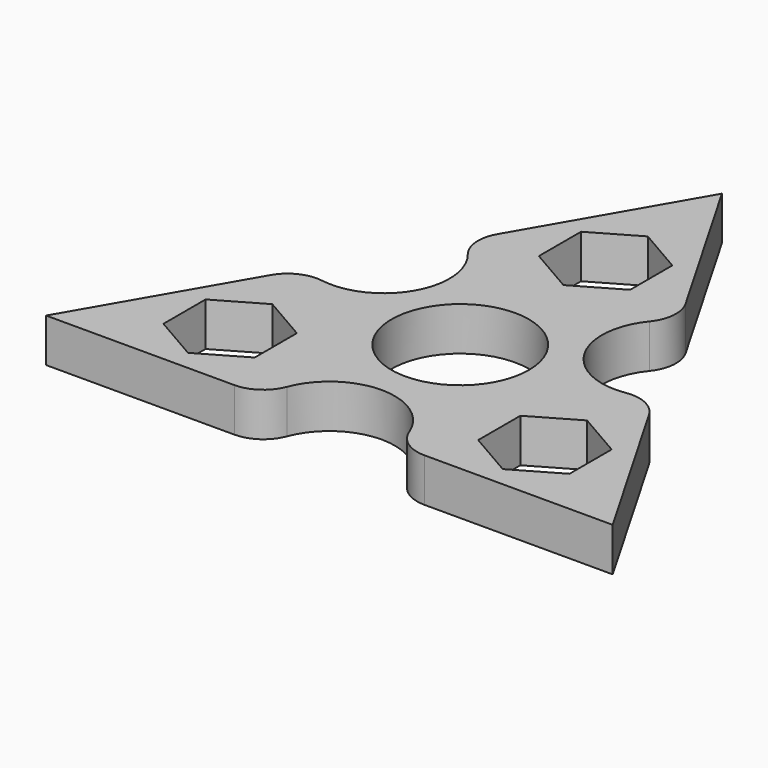
from build123d import *

# Parameters (mm, degrees)
F0_R     = 9.45
F1_DEPTH = 6
F2_R     = 5


with BuildPart() as f1:
    # F0 (on Top) → F1 (new body)
    with BuildSketch(Plane.XY):
        with BuildLine():
            Line((14.9855715851, 19.0442286341), (0, 45))
            Line((0, 45), (-14.9855715851, 19.0442286341))
            ThreePointArc((-14.9855715851, 19.0442286341), (-11.6913429511, 6.75), (-23.9855715851, 3.4557713659))
            Line((-23.9855715851, 3.4557713659), (-38.9711431703, -22.5))
            Line((-38.9711431703, -22.5), (-9, -22.5))
            ThreePointArc((-9, -22.5), (0, -13.5), (9, -22.5))
            Line((9, -22.5), (38.9711431703, -22.5))
            Line((38.9711431703, -22.5), (23.9855715851, 3.4557713659))
            ThreePointArc((23.9855715851, 3.4557713659), (11.6913429511, 6.75), (14.9855715851, 19.0442286341))
        make_face()
        Polygon((-15.3719509172, -16.125), (-21.6506350946, -19.75), (-27.929319272, -16.125), (-27.929319272, -8.875), (-21.6506350946, -5.25), (-15.3719509172, -8.875), align=None, mode=Mode.SUBTRACT)
        Polygon((21.6506350946, -5.25), (27.929319272, -8.875), (27.929319272, -16.125), (21.6506350946, -19.75), (15.3719509172, -16.125), (15.3719509172, -8.875), align=None, mode=Mode.SUBTRACT)
        Circle(F0_R, mode=Mode.SUBTRACT)
        Polygon((-6.2786841774, 28.625), (0, 32.25), (6.2786841774, 28.625), (6.2786841774, 21.375), (0, 17.75), (-6.2786841774, 21.375), align=None, mode=Mode.SUBTRACT)
    extrude(amount=F1_DEPTH)

    # F2
    f2_edges = [f1.edges().sort_by_distance(p)[0] for p in [
        (14.985572, 19.044229, 3),
        (-23.985572, 3.455771, 3),
        (9, -22.5, 3),
        (-14.985572, 19.044229, 3),
        (-9, -22.5, 3),
        (23.985572, 3.455771, 3),
    ]]
    fillet(f2_edges, radius=F2_R)


solid = f1.part
